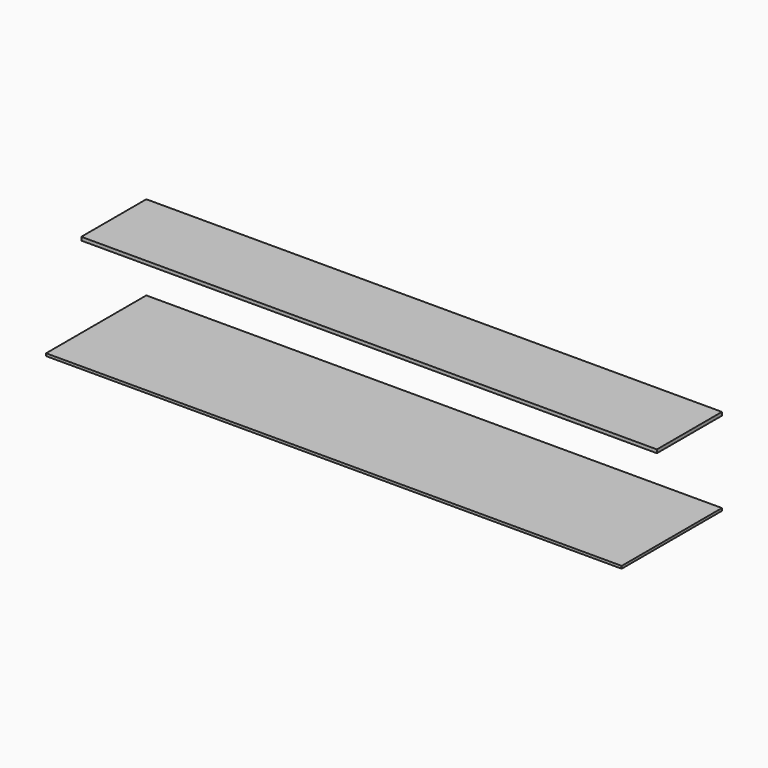
from build123d import *

# Parameters (mm, degrees)
F0_W     = 4318
F0_H     = 939.8
F1_DEPTH = 19.05
F7_W     = 4318
F7_H     = 609.6
F8_DEPTH = 25.4


# Not quite as in the source:
# - the program builds the solid bodies; features that only make, move or delete a surface that nothing else refers to are left out


with BuildPart() as f1:
    # F0 (on Top) → F1 (new body)
    with BuildSketch(Plane.XY):
        Rectangle(F0_W, F0_H)
    extrude(amount=F1_DEPTH)


with BuildPart() as f8:
    # F7 (on offset) → F8 (new body)
    with BuildSketch(Plane.XY.offset(628.65)):
        with Locations((0, 165.1)):
            Rectangle(F7_W, F7_H)
    extrude(amount=F8_DEPTH)


solid = Compound([f1.part, f8.part])
